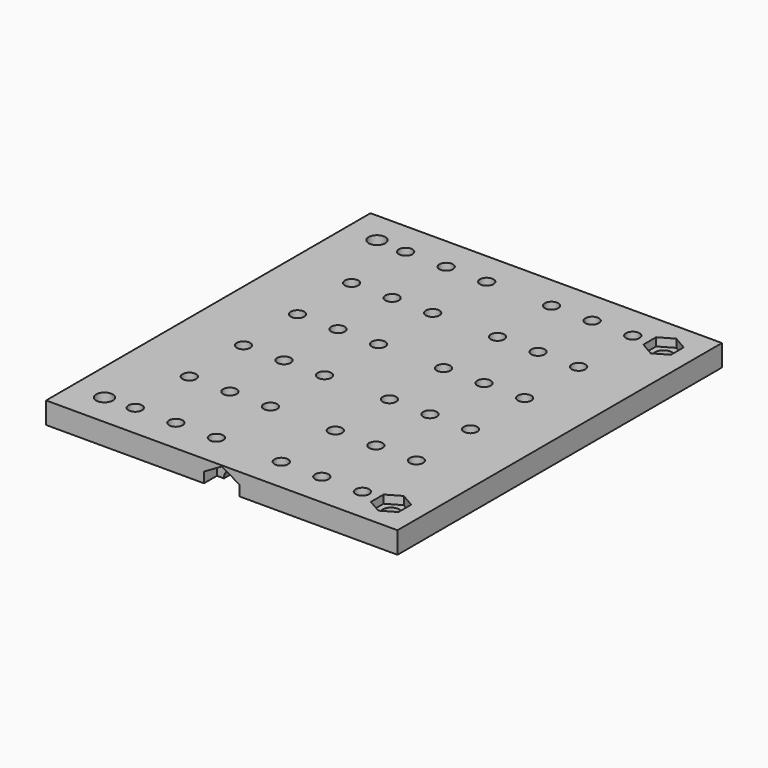
from build123d import *

# Parameters (mm, degrees)
F0_W     = 130
F0_H     = 150
F0_R     = 3.1
F0_R_2   = 2.5
F1_DEPTH = 8
F2_START = 5
F2_DEPTH = 20
F4_DEPTH = 150.001
F5_DEPTH = 6


# Not quite as in the source:
# - a pattern or mirror of a feature is missing from the dataset's text; its kind, count and spacing are read off the source's solid


with BuildPart() as f1:
    # F0 (on Top) → F1 (new body)
    with BuildSketch(Plane.XY):
        Rectangle(F0_W, F0_H)
        with Locations((-53, -63)):
            Circle(F0_R, mode=Mode.SUBTRACT)
        with Locations((-42, -62.5)):
            Circle(F0_R_2, mode=Mode.SUBTRACT)
        with Locations((-27, -62.5)):
            Circle(F0_R_2, mode=Mode.SUBTRACT)
        with Locations((-12, -62.5)):
            Circle(F0_R_2, mode=Mode.SUBTRACT)
        with Locations((-42, -37.5)):
            Circle(F0_R_2, mode=Mode.SUBTRACT)
        with Locations((-42, -12.5)):
            Circle(F0_R_2, mode=Mode.SUBTRACT)
        with Locations((-27, -37.5)):
            Circle(F0_R_2, mode=Mode.SUBTRACT)
        with Locations((-12, -37.5)):
            Circle(F0_R_2, mode=Mode.SUBTRACT)
        with Locations((-27, -12.5)):
            Circle(F0_R_2, mode=Mode.SUBTRACT)
        with Locations((-12, -12.5)):
            Circle(F0_R_2, mode=Mode.SUBTRACT)
        with Locations((12, -62.5)):
            Circle(F0_R_2, mode=Mode.SUBTRACT)
        with Locations((27, -62.5)):
            Circle(F0_R_2, mode=Mode.SUBTRACT)
        with Locations((42, -62.5)):
            Circle(F0_R_2, mode=Mode.SUBTRACT)
        Polygon((53, -57.1110272543), (58.1, -60.0555136271), (58.1, -65.9444863729), (53, -68.8889727457), (47.9, -65.9444863729), (47.9, -60.0555136271), align=None, mode=Mode.SUBTRACT)
        with Locations((12, -37.5)):
            Circle(F0_R_2, mode=Mode.SUBTRACT)
        with Locations((27, -37.5)):
            Circle(F0_R_2, mode=Mode.SUBTRACT)
        with Locations((12, -12.5)):
            Circle(F0_R_2, mode=Mode.SUBTRACT)
        with Locations((27, -12.5)):
            Circle(F0_R_2, mode=Mode.SUBTRACT)
        with Locations((42, -37.5)):
            Circle(F0_R_2, mode=Mode.SUBTRACT)
        with Locations((42, -12.5)):
            Circle(F0_R_2, mode=Mode.SUBTRACT)
        with Locations((-42, 12.5)):
            Circle(F0_R_2, mode=Mode.SUBTRACT)
        with Locations((-27, 12.5)):
            Circle(F0_R_2, mode=Mode.SUBTRACT)
        with Locations((-12, 12.5)):
            Circle(F0_R_2, mode=Mode.SUBTRACT)
        with Locations((-42, 37.5)):
            Circle(F0_R_2, mode=Mode.SUBTRACT)
        with Locations((-53, 63)):
            Circle(F0_R, mode=Mode.SUBTRACT)
        with Locations((-42, 62.5)):
            Circle(F0_R_2, mode=Mode.SUBTRACT)
        with Locations((-27, 37.5)):
            Circle(F0_R_2, mode=Mode.SUBTRACT)
        with Locations((-12, 37.5)):
            Circle(F0_R_2, mode=Mode.SUBTRACT)
        with Locations((-27, 62.5)):
            Circle(F0_R_2, mode=Mode.SUBTRACT)
        with Locations((-12, 62.5)):
            Circle(F0_R_2, mode=Mode.SUBTRACT)
        with Locations((12, 12.5)):
            Circle(F0_R_2, mode=Mode.SUBTRACT)
        with Locations((27, 12.5)):
            Circle(F0_R_2, mode=Mode.SUBTRACT)
        with Locations((42, 12.5)):
            Circle(F0_R_2, mode=Mode.SUBTRACT)
        with Locations((12, 37.5)):
            Circle(F0_R_2, mode=Mode.SUBTRACT)
        with Locations((27, 37.5)):
            Circle(F0_R_2, mode=Mode.SUBTRACT)
        with Locations((12, 62.5)):
            Circle(F0_R_2, mode=Mode.SUBTRACT)
        with Locations((27, 62.5)):
            Circle(F0_R_2, mode=Mode.SUBTRACT)
        with Locations((42, 37.5)):
            Circle(F0_R_2, mode=Mode.SUBTRACT)
        with Locations((42, 62.5)):
            Circle(F0_R_2, mode=Mode.SUBTRACT)
        Polygon((58.1, 65.9444863729), (58.1, 60.0555136271), (53, 57.1110272543), (47.9, 60.0555136271), (47.9, 65.9444863729), (53, 68.8889727457), align=None, mode=Mode.SUBTRACT)
        Polygon((53, 57.1110272543), (58.1, 60.0555136271), (58.1, 65.9444863729), (53, 68.8889727457), (47.9, 65.9444863729), (47.9, 60.0555136271), align=None)
        with Locations((53, 63)):
            Circle(F0_R, mode=Mode.SUBTRACT)
        Polygon((58.1, -65.9444863729), (58.1, -60.0555136271), (53, -57.1110272543), (47.9, -60.0555136271), (47.9, -65.9444863729), (53, -68.8889727457), align=None)
        with Locations((53, -63)):
            Circle(F0_R, mode=Mode.SUBTRACT)
    extrude(amount=F1_DEPTH)

    # F0 (on Top) → F2 (cut)
    with BuildSketch(Plane.XY.offset(F2_START)):
        Polygon((53, 57.1110272543), (58.1, 60.0555136271), (58.1, 65.9444863729), (53, 68.8889727457), (47.9, 65.9444863729), (47.9, 60.0555136271), align=None)
        with Locations((53, 63)):
            Circle(F0_R, mode=Mode.SUBTRACT)
        Polygon((58.1, -65.9444863729), (58.1, -60.0555136271), (53, -57.1110272543), (47.9, -60.0555136271), (47.9, -65.9444863729), (53, -68.8889727457), align=None)
        with Locations((53, -63)):
            Circle(F0_R, mode=Mode.SUBTRACT)
    extrude(amount=F2_DEPTH, mode=Mode.SUBTRACT)

    # F3 (on face) → F4 (cut, through all)
    with BuildSketch(Plane.XZ.offset(75)):
        with BuildLine():
            Line((-4, 0), (4, 0))
            ThreePointArc((4, 0), (0, 4), (-4, 0))
        make_face()
    extrude(amount=-F4_DEPTH, mode=Mode.SUBTRACT)

    # F3 (on face) → F5 (cut)
    with BuildSketch(Plane.XZ.offset(75)):
        with BuildLine():
            Line((6.6, 0), (4, 0))
            ThreePointArc((4, 0), (0, -4), (-4, 0))
            Line((-4, 0), (-6.6, 0))
            Line((-6.6, 0), (-6.6, -3.8105117767))
            Line((-6.6, -3.8105117767), (0, -7.6210235533))
            Line((0, -7.6210235533), (6.6, -3.8105117767))
            Line((6.6, -3.8105117767), (6.6, 0))
        make_face()
        with BuildLine():
            ThreePointArc((-4, 0), (0, 4), (4, 0))
            Line((4, 0), (6.6, 0))
            Line((6.6, 0), (6.6, 3.8105117767))
            Line((6.6, 3.8105117767), (0, 7.6210235533))
            Line((0, 7.6210235533), (-6.6, 3.8105117767))
            Line((-6.6, 3.8105117767), (-6.6, 0))
            Line((-6.6, 0), (-4, 0))
        make_face()
    f5 = extrude(amount=-F5_DEPTH, mode=Mode.SUBTRACT)

    # F5_copies: F5 across plane
    add(f5.mirror(Plane.ZX), mode=Mode.SUBTRACT)


solid = f1.part
